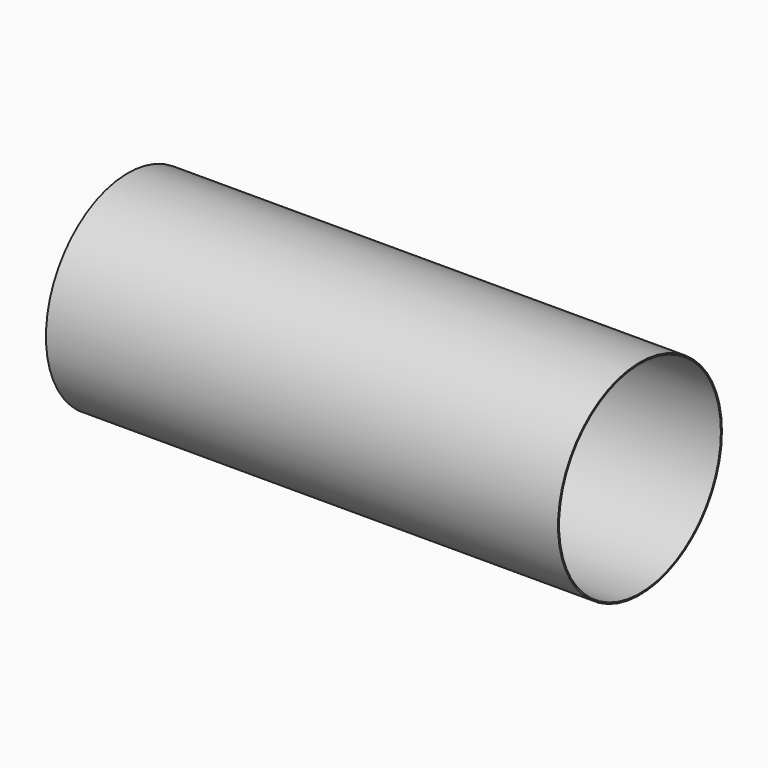
from build123d import *

# Parameters (mm, degrees)
F0_R     = 2000
F0_R_2   = 1975
F1_DEPTH = 10000


# Not quite as in the source:
# - a feature of the source that left no trace in its solid (it failed there, or was rolled back) is left out


with BuildPart() as f1:
    # F0 (on Right) → F1 (new body)
    with BuildSketch(Plane.YZ):
        Circle(F0_R)
        Circle(F0_R_2, mode=Mode.SUBTRACT)
    extrude(amount=F1_DEPTH)


solid = f1.part
